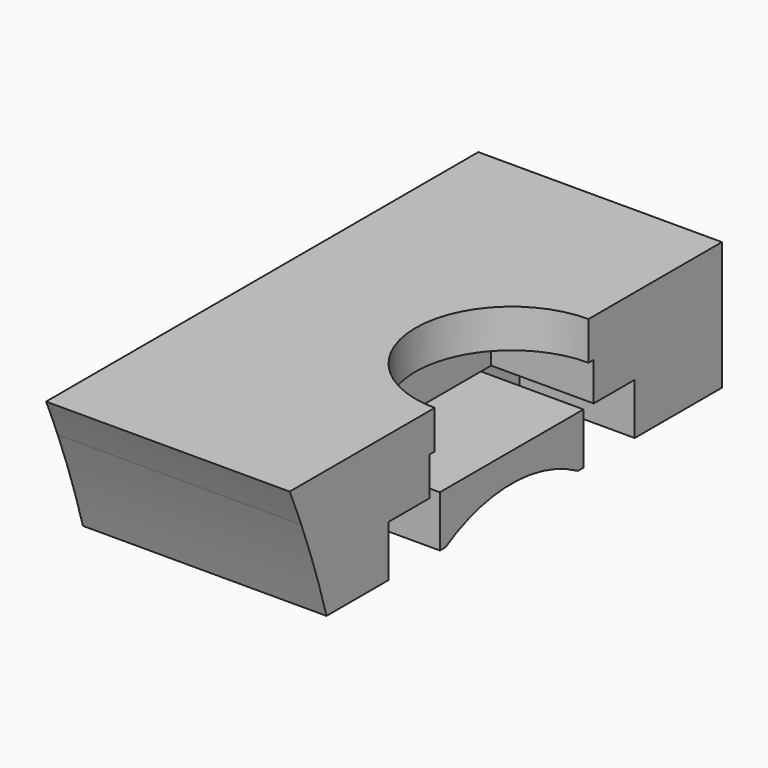
from build123d import *

# Parameters (mm, degrees)
F0_W      = 22
F0_H      = 10
F1_DEPTH  = 19
F2_W      = 19
F2_H      = 19
F3_DEPTH  = 10
F4_W      = 9
F4_H      = 5
F5_DEPTH  = 4
F7_DEPTH  = 25
F9_DEPTH  = 19
F10_DEPTH = 25
F12_DEPTH = 10
F14_DEPTH = 8
F16_DEPTH = 3


# Not quite as in the source:
# - a feature names something its author has since deleted; it is built from what else it names


with BuildPart() as f1:
    # F0 (on Right) → F1 (new body)
    with BuildSketch(Plane.YZ):
        with Locations((10.6502909437, -9.5214466426)):
            Rectangle(F0_W, F0_H)
    extrude(amount=F1_DEPTH)

    # F2 (on face) → F3 (join)
    with BuildSketch(Plane.XY.offset(-4.5214466426)):
        with Locations((9.5, -9.8497090563)):
            Rectangle(F2_W, F2_H)
    extrude(amount=-F3_DEPTH)

    # F4 (on face) → F5 (cut)
    with BuildSketch(Plane(origin=(0, 0, -14.5214466426), x_dir=(1, 0, 0), z_dir=(0, 0, -1))):
        with Locations((14.5, 8.3497090563)):
            Rectangle(F4_W, F4_H)
        with Locations((14.5, -10.6502909437)):
            Rectangle(F4_W, F4_H)
    extrude(amount=-F5_DEPTH, mode=Mode.SUBTRACT)

    # F6 (on face) → F7 (cut)
    with BuildSketch(Plane(origin=(0, 0, 0), x_dir=(0, -1, 0), z_dir=(-1, 0, 0))):
        with BuildLine():
            Line((-7.5971894228, -14.5214466426), (5.2966075354, -14.5214466426))
            ThreePointArc((5.2966075354, -14.5214466426), (-1.1502909437, -12.7714466426), (-7.5971894228, -14.5214466426))
        make_face()
        with BuildLine():
            ThreePointArc((-7.5971894228, -14.5214466426), (-7.4892397679, -36.5840063737), (11.5997090563, -25.5214466426))
            ThreePointArc((11.5997090563, -25.5214466426), (9.9122687874, -19.1824978184), (5.2966075354, -14.5214466426))
            Line((5.2966075354, -14.5214466426), (-7.5971894228, -14.5214466426))
        make_face()
    extrude(amount=-F7_DEPTH, mode=Mode.SUBTRACT)

    # F8 (on face) → F9 (join)
    with BuildSketch(Plane(origin=(0, 0, 0), x_dir=(0, -1, 0), z_dir=(-1, 0, 0))):
        with BuildLine():
            ThreePointArc((19.3497090563, -7.2717528529), (78.9260517523, -115.1245254627), (173.8108090563, -36.5214466426))
            ThreePointArc((173.8108090563, -36.5214466426), (110.1555805515, 41.7910583919), (20.489597937, -4.5214466426))
            Line((20.489597937, -4.5214466426), (33.1326909363, -4.5214466426))
            Line((33.1326909363, -4.5214466426), (33.1326909363, -14.5214466426))
            Line((33.1326909363, -14.5214466426), (19.3497090563, -14.5214466426))
            Line((19.3497090563, -14.5214466426), (19.3497090563, -7.2717528529))
        make_face()
        with BuildLine():
            ThreePointArc((19.3497090563, -7.2717528529), (19.9068584447, -5.8912967246), (20.489597937, -4.5214466426))
            Line((20.489597937, -4.5214466426), (19.3497090563, -4.5214466426))
            Line((19.3497090563, -4.5214466426), (19.3497090563, -7.2717528529))
        make_face()
    extrude(amount=-F9_DEPTH)

    # F8 (on face) → F10 (cut)
    with BuildSketch(Plane(origin=(0, 0, 0), x_dir=(0, -1, 0), z_dir=(-1, 0, 0))):
        with BuildLine():
            ThreePointArc((19.3497090563, -7.2717528529), (78.9260517523, -115.1245254627), (173.8108090563, -36.5214466426))
            ThreePointArc((173.8108090563, -36.5214466426), (110.1555805515, 41.7910583919), (20.489597937, -4.5214466426))
            Line((20.489597937, -4.5214466426), (33.1326909363, -4.5214466426))
            Line((33.1326909363, -4.5214466426), (33.1326909363, -14.5214466426))
            Line((33.1326909363, -14.5214466426), (19.3497090563, -14.5214466426))
            Line((19.3497090563, -14.5214466426), (19.3497090563, -7.2717528529))
        make_face()
    extrude(amount=-F10_DEPTH, mode=Mode.SUBTRACT)

    # F11 (on face) → F12 (join)
    with BuildSketch(Plane(origin=(0, 0, 0), x_dir=(0, -1, 0), z_dir=(-1, 0, 0))):
        with BuildLine():
            ThreePointArc((-10.6762534344, -17.046864728), (-9.2359267268, -15.6632016678), (-7.5971894228, -14.5214466426))
            Line((-7.5971894228, -14.5214466426), (-21.6502909437, -14.5214466426))
            Line((-21.6502909437, -14.5214466426), (-21.6502909437, -18.9818836282))
            Line((-21.6502909437, -18.9818836282), (-10.6762534344, -17.046864728))
        make_face()
    extrude(amount=-F12_DEPTH)

    # F13 (on face) → F14 (cut)
    with BuildSketch(Plane.YZ.offset(19)):
        Polygon((1.1502909437, -4.5214466426), (-6.8497090563, -4.5214466426), (-6.8497090563, -10.5214466426), (-5.8497090563, -10.5214466426), (1.1502909437, -10.5214466426), align=None)
        Polygon((9.1502909437, -4.5214466426), (1.1502909437, -4.5214466426), (1.1502909437, -10.5214466426), (8.1502909437, -10.5214466426), (9.1502909437, -10.5214466426), align=None)
    extrude(amount=-F14_DEPTH, mode=Mode.SUBTRACT)

    # F15 (on face) → F16 (join)
    with BuildSketch(Plane.XY.offset(-4.5214466426)):
        with BuildLine():
            ThreePointArc((19, -6.3497090563), (11.5, 1.1502909437), (19, 8.6502909437))
            Line((19, 8.6502909437), (19, 9.1502909437))
            Line((19, 9.1502909437), (11, 9.1502909437))
            Line((11, 9.1502909437), (11, -6.8497090563))
            Line((11, -6.8497090563), (19, -6.8497090563))
            Line((19, -6.8497090563), (19, -6.3497090563))
        make_face()
    extrude(amount=-F16_DEPTH)


solid = f1.part
